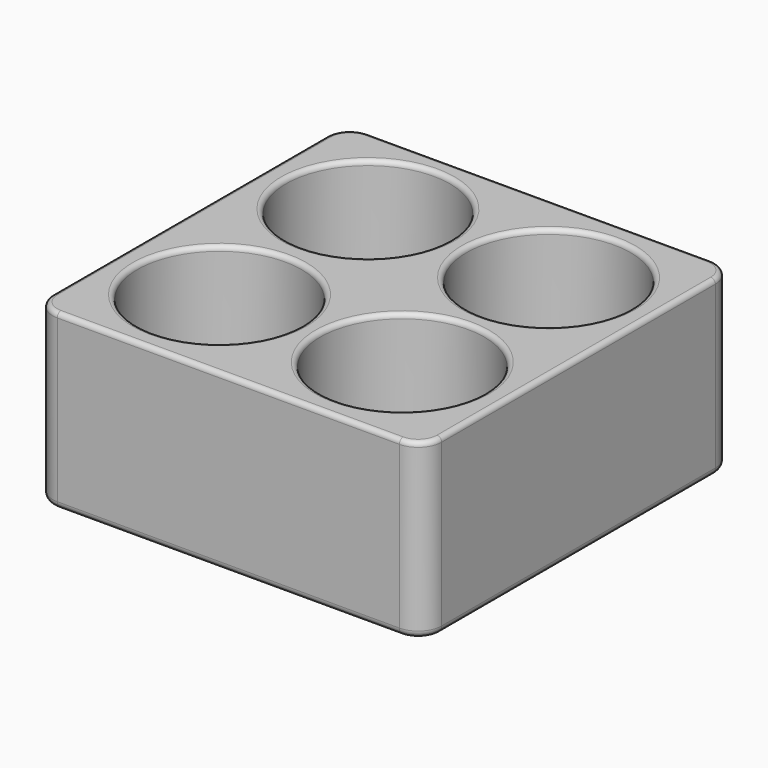
from build123d import *

# Parameters (mm, degrees)
F0_W         = 83
F0_H         = 83
F0_R         = 17.5
F1_DEPTH     = 36
F2_R         = 1
F3_W         = 83
F3_H         = 83
F4_DEPTH     = 1
F5_T1_DEPTH  = 49.5
F5_T4_ANGLE  = 90
F5_T6_ANGLE  = 90
F5_T8_ANGLE  = 90
F5_T10_ANGLE = 90
F6_R         = 1.5


# Not quite as in the source:
# - a fillet or chamfer that OpenCascade refuses, or shapes differently, is made with other operations: its cross-section is extruded or revolved along the edge and cut away or added
# - a feature names something its author has since deleted; it is built from what else it names


with BuildPart() as f1:
    # F0 (on Top) → F1 (new body)
    with BuildSketch(Plane.XY):
        with Locations((-3, 19.5)):
            Rectangle(F0_W, F0_H)
        with Locations((-22.5, 0)):
            Circle(F0_R, mode=Mode.SUBTRACT)
        with Locations((16.5, 0)):
            Circle(F0_R, mode=Mode.SUBTRACT)
        with Locations((-22.5, 39.5840890706)):
            Circle(F0_R, mode=Mode.SUBTRACT)
        with Locations((16.5, 39)):
            Circle(F0_R, mode=Mode.SUBTRACT)
    extrude(amount=F1_DEPTH)

    # F2
    f2_edges = [f1.edges().sort_by_distance(p)[0] for p in [
        (-3, 61, 36),
        (-44.5, 19.5, 36),
        (-3, -22, 36),
        (38.5, 19.5, 36),
        (-40, 0, 36),
        (-1, 0, 36),
        (-40, 39.584089, 36),
        (-1, 39, 36),
    ]]
    fillet(f2_edges, radius=F2_R)

    # F3 (on face) → F4 (join)
    with BuildSketch(Plane(origin=(0, 0, 0), x_dir=(1, 0, 0), z_dir=(0, 0, -1))):
        with Locations((-3, -19.5)):
            Rectangle(F3_W, F3_H)
    extrude(amount=F4_DEPTH)

    # F5: fillet of radius 5 on 4 edges, made by hand

    # F5_s2 → F5_t1 (cut)
    with BuildSketch(Plane.XY.offset(-13.5)):
        with BuildLine():
            ThreePointArc((-39.5, 61), (-43.0355339059, 59.5355339059), (-44.5, 56))
            Line((-44.5, 56), (-44.5, 61))
            Line((-44.5, 61), (-39.5, 61))
        make_face()
        with BuildLine():
            ThreePointArc((-39.5, -22), (-43.0355339059, -20.5355339059), (-44.5, -17))
            Line((-44.5, -17), (-44.5, -22))
            Line((-44.5, -22), (-39.5, -22))
        make_face()
        with BuildLine():
            ThreePointArc((33.5, -22), (37.0355339059, -20.5355339059), (38.5, -17))
            Line((38.5, -17), (38.5, -22))
            Line((38.5, -22), (33.5, -22))
        make_face()
        with BuildLine():
            ThreePointArc((33.5, 61), (37.0355339059, 59.5355339059), (38.5, 56))
            Line((38.5, 56), (38.5, 61))
            Line((38.5, 61), (33.5, 61))
        make_face()
    extrude(amount=F5_T1_DEPTH, mode=Mode.SUBTRACT)

    # F5_s3 → F5_t4 (revolve, cut)
    with BuildSketch(Plane.XZ.offset(-56)):
        with BuildLine():
            ThreePointArc((37.5, 36), (38.2071067812, 35.7071067812), (38.5, 35))
            Line((38.5, 35), (38.5, 36))
            Line((38.5, 36), (37.5, 36))
        make_face()
    revolve(axis=Axis((33.5, 56, 36), (0, 0, 1)), revolution_arc=F5_T4_ANGLE, mode=Mode.SUBTRACT)

    # F5_s5 → F5_t6 (revolve, cut)
    with BuildSketch(Plane.YZ.offset(33.5)):
        with BuildLine():
            ThreePointArc((-21, 36), (-21.7071067812, 35.7071067812), (-22, 35))
            Line((-22, 35), (-22, 36))
            Line((-22, 36), (-21, 36))
        make_face()
    revolve(axis=Axis((33.5, -17, 36), (0, 0, 1)), revolution_arc=F5_T6_ANGLE, mode=Mode.SUBTRACT)

    # F5_s7 → F5_t8 (revolve, cut)
    with BuildSketch(Plane.XZ.offset(17)):
        with BuildLine():
            ThreePointArc((-43.5, 36), (-44.2071067812, 35.7071067812), (-44.5, 35))
            Line((-44.5, 35), (-44.5, 36))
            Line((-44.5, 36), (-43.5, 36))
        make_face()
    revolve(axis=Axis((-39.5, -17, 36), (0, 0, 1)), revolution_arc=F5_T8_ANGLE, mode=Mode.SUBTRACT)

    # F5_s9 → F5_t10 (revolve, cut)
    with BuildSketch(Plane.YZ.offset(-39.5)):
        with BuildLine():
            ThreePointArc((60, 36), (60.7071067812, 35.7071067812), (61, 35))
            Line((61, 35), (61, 36))
            Line((61, 36), (60, 36))
        make_face()
    revolve(axis=Axis((-39.5, 56, 36), (0, 0, 1)), revolution_arc=F5_T10_ANGLE, mode=Mode.SUBTRACT)

    # F6
    f6_edges = [f1.edges().sort_by_distance(p)[0] for p in [
        (37.035534, -20.535534, -1),
        (38.5, 19.5, -1),
        (37.035534, 59.535534, -1),
        (-3, 61, -1),
        (-43.035534, 59.535534, -1),
        (-44.5, 19.5, -1),
        (-43.035534, -20.535534, -1),
        (-3, -22, -1),
    ]]
    fillet(f6_edges, radius=F6_R)


solid = f1.part
